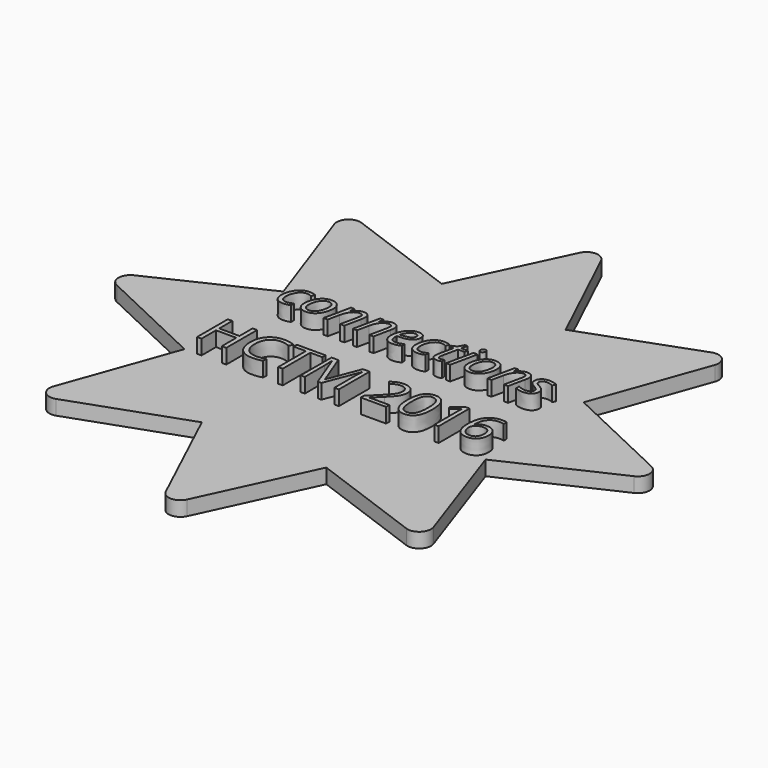
from build123d import *

# Parameters (mm, degrees)
F1_DEPTH       = 3.175
F2_TEXT_SIZE   = 10.8870005028
F2_TEXT_SIZE_2 = 11.6128034683
F3_DEPTH       = 3.175
F4_R           = 2.54


# Not quite as in the source:
# - Text() gives the source's letters only with a copy of the font that has no kerning and outlines rounded to 1/6400 em; it was checked with that copy


with BuildPart() as f1:
    # F0 (on Top) → F1 (new body)
    with BuildSketch(Plane.XY):
        Polygon((-28.3609493054, 67.0965386089), (-41.7351698852, 95.3289603349), (-55.0685268245, 67.1290343162), (-84.546243248, 77.9178810772), (-74.1111314273, 48.3222508337), (-102.2918312228, 34.9411179777), (-73.9932222641, 21.5564814862), (-84.5462469733, -7.8622812871), (-55.0685286871, 2.5728305336), (-41.7351698852, -25.8415641729), (-28.4477196983, 2.7957295533), (0.9382614517, -7.9666527454), (-9.3561908579, 21.7936735135), (18.8673125231, 34.9411179777), (-9.5007581986, 48.3604248147), (1.0582344257, 77.8398474213), align=None)
    extrude(amount=F1_DEPTH)

    # F2 (on face) → F3 (join)
    with BuildSketch(Plane.XY.offset(3.175)):
        with Locations((-70.3265294433, 40.2571596205)):
            Text('connections', F2_TEXT_SIZE, font='Open Sans', font_style=FontStyle.ITALIC, text_align=(TextAlign.LEFT, TextAlign.BOTTOM))
        with Locations((-72.4255376141, 21.5564814862)):
            Text('HCTM 2016', F2_TEXT_SIZE_2, font='Open Sans', text_align=(TextAlign.LEFT, TextAlign.BOTTOM))
    extrude(amount=F3_DEPTH)

    # F4
    f4_edges = [f1.edges().sort_by_distance(p)[0] for p in [
        (-102.291831, 34.941118, 1.5875),
        (-84.546247, -7.862281, 1.5875),
        (-41.73517, -25.841564, 1.5875),
        (0.938261, -7.966653, 1.5875),
        (18.867313, 34.941118, 1.5875),
        (1.058234, 77.839847, 1.5875),
        (-41.73517, 95.32896, 1.5875),
        (-84.546243, 77.917881, 1.5875),
    ]]
    fillet(f4_edges, radius=F4_R)


solid = f1.part
